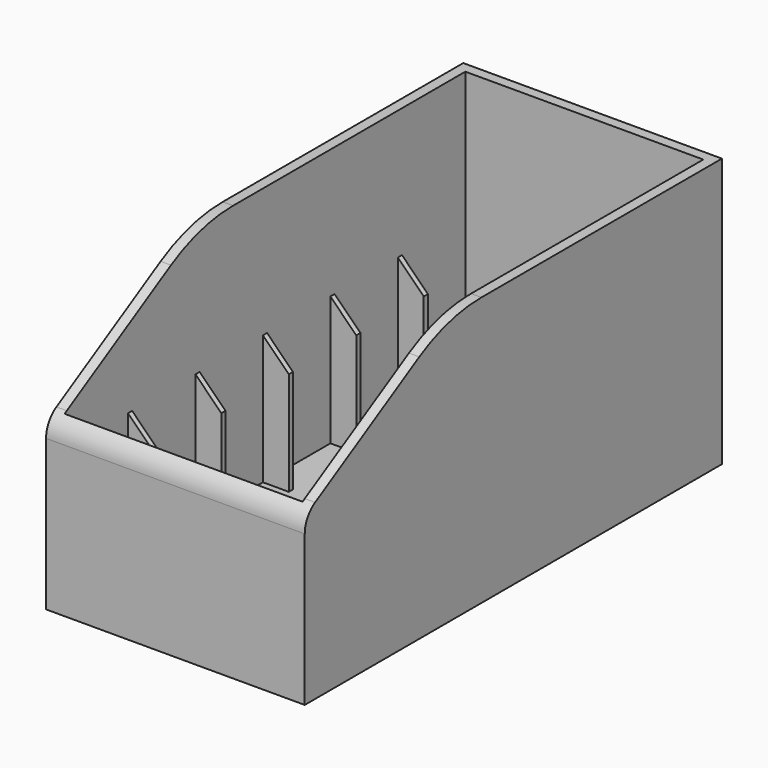
from build123d import *

# Parameters (mm, degrees)
F0_W        = 50
F0_H        = 100.8
F0_W_2      = 46
F0_H_2      = 96.8
F1_DEPTH    = 50
F2_W        = 50
F2_H        = 100.8
F2_W_2      = 26
F2_H_2      = 76.8
F3_DEPTH    = 2
F4_T1_DEPTH = 229.2385588234
F5_R        = 30
F6_T1_DEPTH = 64.4337567297
F7_R        = 5
F8_W        = 5
F8_H        = 1
F9_DEPTH    = 25
F10_SIZE    = 4.99999


# Not quite as in the source:
# - a fillet or chamfer that OpenCascade refuses, or shapes differently, is made with other operations: its cross-section is extruded or revolved along the edge and cut away or added
# - a fillet or chamfer is up to 0.001 mm smaller than in the source, because OpenCascade refuses the exact size


with BuildPart() as f1:
    # F0 (on Top) → F1 (new body)
    with BuildSketch(Plane.XY):
        Rectangle(F0_W, F0_H)
        Rectangle(F0_W_2, F0_H_2, mode=Mode.SUBTRACT)
    extrude(amount=F1_DEPTH)

    # F2 (on Top) → F3 (join)
    with BuildSketch(Plane.XY):
        Rectangle(F2_W, F2_H)
        Rectangle(F2_W_2, F2_H_2, mode=Mode.SUBTRACT)
    extrude(amount=-F3_DEPTH)

    # F4: chamfer of 20 x 34.6410161514 on 1 edges, made by hand

    # F4_s2 → F4_t1 (cut)
    with BuildSketch(Plane.YZ.offset(-114.6192794117)):
        Polygon((-15.7589838486, 50), (-50.4, 30), (-50.4, 50), align=None)
    extrude(amount=F4_T1_DEPTH, mode=Mode.SUBTRACT)

    # F5
    f5_edges = [f1.edges().sort_by_distance(p)[0] for p in [
        (24, -15.758984, 50),
        (-24, -15.758984, 50),
    ]]
    fillet(f5_edges, radius=F5_R)

    # F6: fillet of radius 5 on 1 edges, made by hand

    # F6_s2 → F6_t1 (cut)
    with BuildSketch(Plane.YZ.offset(-32.2168783649)):
        with BuildLine():
            ThreePointArc((-47.9, 31.443375673), (-49.7301270189, 29.6132486541), (-50.4, 27.1132486541))
            Line((-50.4, 27.1132486541), (-50.4, 30))
            Line((-50.4, 30), (-47.9, 31.443375673))
        make_face()
    extrude(amount=F6_T1_DEPTH, mode=Mode.SUBTRACT)

    # F7
    f7_edges = [f1.edges().sort_by_distance(p)[0] for p in [
        (13, 38.4, -1),
        (-13, 38.4, -1),
        (13, -38.4, -1),
        (-13, -38.4, -1),
    ]]
    fillet(f7_edges, radius=F7_R)

    # F8 (on face) → F9 (join)
    with BuildSketch(Plane.XY):
        with Locations((-20.5, 32.6)):
            Rectangle(F8_W, F8_H)
        with Locations((-20.5, 16.3)):
            Rectangle(F8_W, F8_H)
        with Locations((-20.5, 0)):
            Rectangle(F8_W, F8_H)
        with Locations((-20.5, -16.3)):
            Rectangle(F8_W, F8_H)
        with Locations((-20.5, -32.6)):
            Rectangle(F8_W, F8_H)
        with Locations((20.5, -32.6)):
            Rectangle(F8_W, F8_H)
        with Locations((20.5, -16.3)):
            Rectangle(F8_W, F8_H)
        with Locations((20.5, 16.3)):
            Rectangle(F8_W, F8_H)
        with Locations((20.5, 0)):
            Rectangle(F8_W, F8_H)
        with Locations((20.5, 32.6)):
            Rectangle(F8_W, F8_H)
    extrude(amount=F9_DEPTH)

    # F10 (size 5 in the source; OpenCascade refuses exactly that, so slightly less here)
    f10_edges = [f1.edges().sort_by_distance(p)[0] for p in [
        (-18, 32.6, 25),
        (-18, 16.3, 25),
        (-18, 0, 25),
        (-18, -16.3, 25),
        (-18, -32.6, 25),
        (18, -32.6, 25),
        (18, -16.3, 25),
        (18, 0, 25),
        (18, 16.3, 25),
        (18, 32.6, 25),
    ]]
    chamfer(f10_edges, length=F10_SIZE)


solid = f1.part
